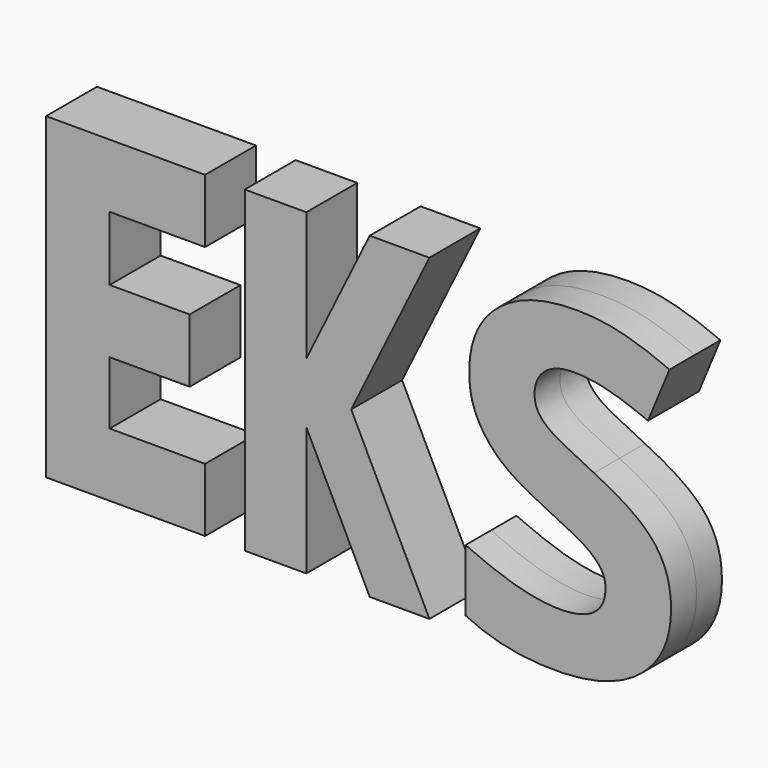
from build123d import *

# Parameters (mm, degrees)
F0_TEXT_SIZE = 176.3888888889
F1_DEPTH     = 12.7


# Not quite as in the source:
# - Text() gives the source's letters only with a copy of the font that has no kerning and outlines rounded to 1/6400 em; it was checked with that copy


with BuildPart() as f1:
    # F0 (on Front) → F1 (new body, symmetric)
    with BuildSketch(Plane.XZ):
        Polygon((-12.2959449618, -63.5), (12.2959449618, -63.5), (12.2959449618, -12.0478673948), (37.604132599, -63.5), (61.4517898217, -63.5), (30.2175176235, 0), (61.4517898217, 63.5), (37.604132599, 63.5), (12.2959449618, 12.0478673948), (12.2959449618, 63.5), (-12.2959449618, 63.5), align=None)
        Polygon((-28.1455449618, 38.1), (-28.1455449618, 63.5), (-91.6455449618, 63.5), (-91.6455449618, -63.5), (-66.2455449618, -63.5), (-28.1455449618, -63.5), (-28.1455449618, -38.1), (-66.2455449618, -38.1), (-66.2455449618, -13.0049362779), (-34.3163563533, -13.0049362779), (-34.3163563533, 12.3950637221), (-66.2455449618, 12.3950637221), (-66.2455449618, 38.1), align=None)
        with Locations((67.7808177405, -63.5)):
            Text('S', F0_TEXT_SIZE, font='Open Sans', font_style=FontStyle.BOLD, text_align=(TextAlign.LEFT, TextAlign.BOTTOM))
    extrude(amount=F1_DEPTH, both=True)


solid = f1.part
